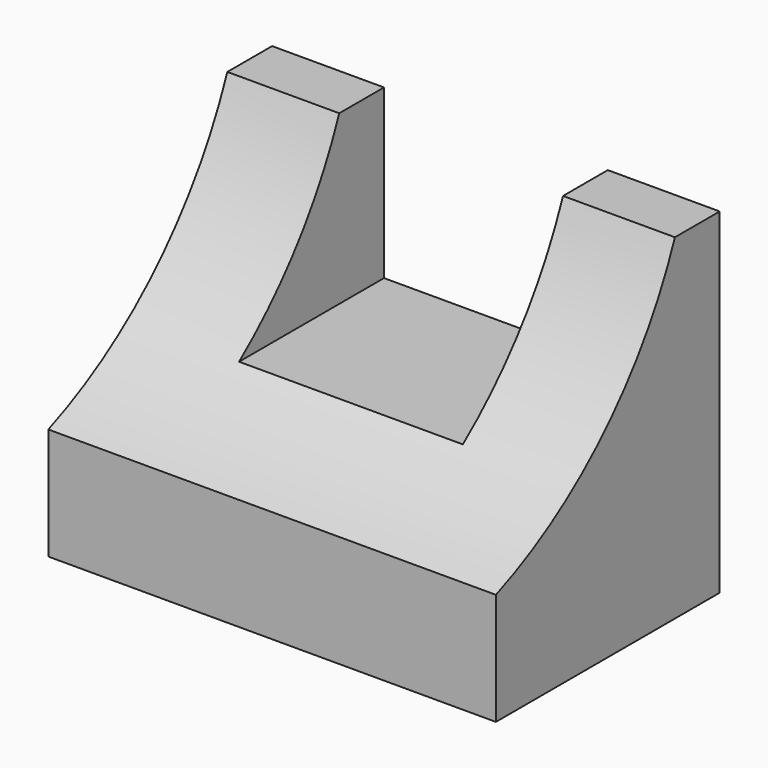
from build123d import *

# Parameters (mm, degrees)
F0_W     = 50.8
F0_H     = 38.1
F1_DEPTH = 31.75
F2_W     = 25.4
F2_H     = 19.05
F3_DEPTH = 19.05
F4_DEPTH = 25.4
F6_DEPTH = 50.8


with BuildPart() as f1:
    # F0 (on Front) → F1 (new body)
    with BuildSketch(Plane.XZ):
        with Locations((-45.1402231145, 19.05)):
            Rectangle(F0_W, F0_H)
    extrude(amount=F1_DEPTH)

    # F2 (on face) → F3 (cut)
    with BuildSketch(Plane.XZ.offset(31.75)):
        with Locations((-45.1402231145, 28.575)):
            Rectangle(F2_W, F2_H)
    extrude(amount=-F3_DEPTH, mode=Mode.SUBTRACT)

    # F4 (cut): a face of the model
    f4_faces = [f1.faces().sort_by_distance(p)[0] for p in [
        (-45.1402231145, -12.7, 28.575),
    ]]
    extrude(f4_faces, amount=-F4_DEPTH, mode=Mode.SUBTRACT)

    # F5 (on face) → F6 (cut)
    with BuildSketch(Plane.YZ.offset(-19.7402231145)):
        with BuildLine():
            ThreePointArc((-31.75, 12.7), (-16.3850971413, 22.7350971413), (-6.35, 38.1))
            Line((-6.35, 38.1), (-31.75, 38.1))
            Line((-31.75, 38.1), (-31.75, 12.7))
        make_face()
    extrude(amount=-F6_DEPTH, mode=Mode.SUBTRACT)


solid = f1.part
